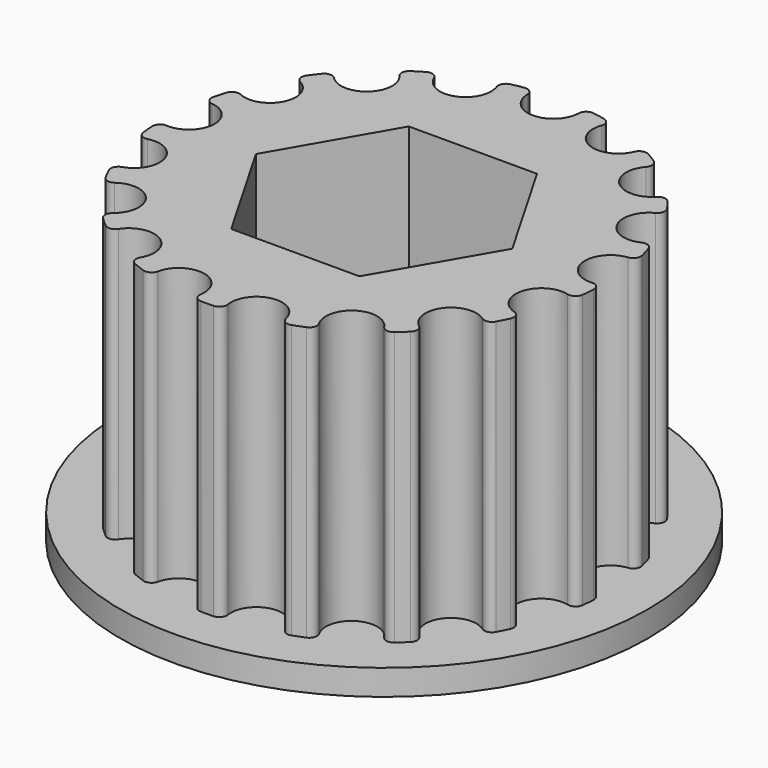
from build123d import *

# Parameters (mm, degrees)
F2_R            = 12.9556701783
F3_DEPTH        = 16
F5_DEPTH        = 16
F5_COPIES_COUNT = 17
F8_R            = 15.4556701783
F8_R_2          = 12.9556701783
F9_DEPTH        = 1.5
F10_DEPTH       = 17.501


# Not quite as in the source:
# - a feature of the source that left no trace in its solid (it failed there, or was rolled back) is left out
# - a pattern or mirror of a feature is missing from the dataset's text; its kind, count and spacing are read off the source's solid


with BuildPart() as f3:
    # F2 (on Top) → F3 (new body)
    with BuildSketch(Plane.XY):
        Circle(F2_R)
    extrude(amount=F3_DEPTH)

    # F4 (on face) → F5 (cut, through all)
    with BuildSketch(Plane.XY.offset(16)):
        with BuildLine():
            ThreePointArc((-2.019679411, 12.797276462), (-1.6609629062, 12.6980751446), (-1.4996370898, 12.362676258))
            ThreePointArc((-1.4996370898, 12.362676258), (0, 10.8956701783), (1.4996370898, 12.362676258))
            ThreePointArc((1.4996370898, 12.362676258), (1.6609629062, 12.6980751446), (2.019679411, 12.797276462))
            ThreePointArc((2.019679411, 12.797276462), (0, 12.9556701783), (-2.019679411, 12.797276462))
        make_face()
    f5 = extrude(amount=-F5_DEPTH, mode=Mode.SUBTRACT)

    # F5_copies: F5 ×17 about axis
    f5_copies_axis = Axis((0, 0, 0), (0, 0, 1))
    for i in range(1, F5_COPIES_COUNT):
        add(f5.rotate(f5_copies_axis, i * 360 / F5_COPIES_COUNT), mode=Mode.SUBTRACT)

    # F8 (on face) + F2 (on Top) → F9 (join)
    with BuildSketch(Plane.XY):
        Circle(F8_R)
        Circle(F8_R_2, mode=Mode.SUBTRACT)
    with BuildSketch(Plane.XY):
        Circle(F2_R)
    extrude(amount=-F9_DEPTH)

    # F7 (on face) → F10 (cut, through all)
    with BuildSketch(Plane.XY.offset(16)):
        Polygon((3.7527767497, 6.5), (-3.7527767497, 6.5), (-7.5055534995, 0), (-3.7527767497, -6.5), (3.7527767497, -6.5), (7.5055534995, 0), align=None)
    extrude(amount=-F10_DEPTH, mode=Mode.SUBTRACT)


solid = f3.part
